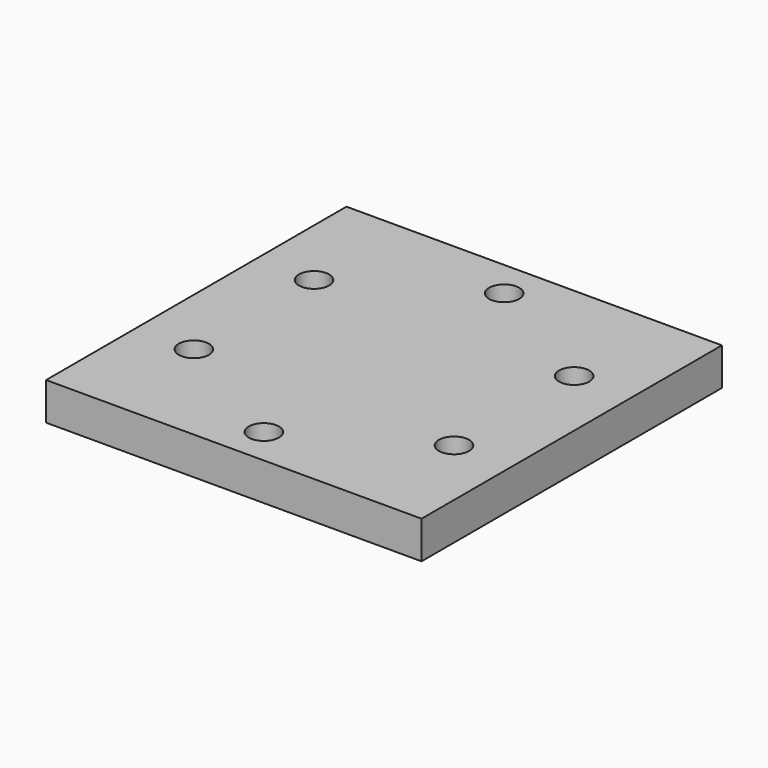
from build123d import *

# Parameters (mm, degrees)
F0_W     = 63.5
F0_H     = 63.5
F1_DEPTH = 6.35
F2_D     = 5.1054
F2_DEPTH = 4.77
F2_TIP   = 1.5338169022


# Not quite as in the source:
# - a length typed as a fraction of an inch, garbled in the dataset ("3 / 203.2 mm" for 3/8 in), is restored


with BuildPart() as f1:
    # F0 (on Top) → F1 (new body)
    with BuildSketch(Plane.XY):
        Rectangle(F0_W, F0_H)
    extrude(amount=-F1_DEPTH)

    # F2
    with Locations(Plane.XY):
        with Locations((0, -25.4), (21.9970452561, -12.7), (21.9970452561, 12.7), (0, 25.4), (-21.9970452561, -12.7), (-21.9970452561, 12.7)):
            Hole(F2_D / 2, depth=F2_DEPTH)
            with Locations((0, 0, -(F2_DEPTH + F2_TIP / 2))):  # 118° drill point
                Cone(0, F2_D / 2, F2_TIP, mode=Mode.SUBTRACT)


solid = f1.part
